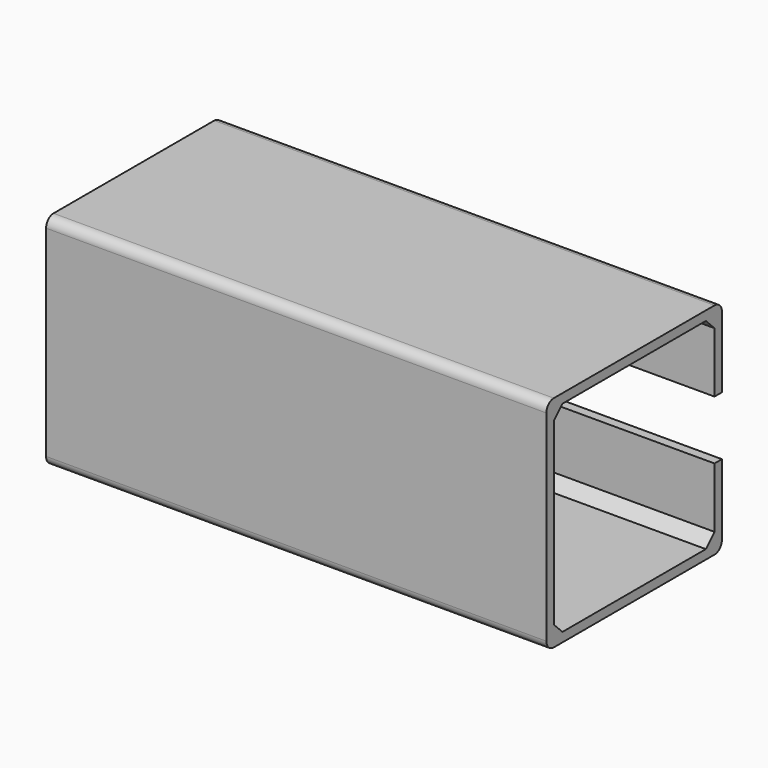
from build123d import *

# Parameters (mm, degrees)
F1_W      = 47.35
F1_H      = 47.35
F2_DEPTH  = 2
F3_DEPTH  = 107.95
F4_R      = 6.35
F7_DEPTH  = 107.951
F8_R      = 6.35
F9_DEPTH  = 25
F10_R     = 2
F11_W     = 2
F11_H     = 12.7
F12_DEPTH = 107.951
F13_DEPTH = 25


# Not quite as in the source:
# - a feature names something its author has since deleted; it is built from what else it names


with BuildPart() as f2:
    # F1 (on Right) → F2 (new body)
    with BuildSketch(Plane.YZ):
        Rectangle(F1_W, F1_H)
        Polygon((19.3428993274, 21.675), (21.675, 21.675), (21.675, 19.3428993274), (21.675, -19.3428993274), (21.675, -21.675), (19.3428993274, -21.675), (-19.3428993274, -21.675), (-21.675, -21.675), (-21.675, -19.3428993274), (-21.675, 19.3428993274), (-21.675, 21.675), (-19.3428993274, 21.675), align=None, mode=Mode.SUBTRACT)
        Polygon((21.675, 19.3428993274), (19.3428993274, 21.675), (-19.3428993274, 21.675), (-21.675, 19.3428993274), (-21.675, -19.3428993274), (-19.3428993274, -21.675), (19.3428993274, -21.675), (21.675, -19.3428993274), align=None)
        Polygon((-19.3428993274, -21.675), (-21.675, -19.3428993274), (-21.675, -21.675), align=None)
        Polygon((21.675, -21.675), (21.675, -19.3428993274), (19.3428993274, -21.675), align=None)
        Polygon((21.675, 19.3428993274), (21.675, 21.675), (19.3428993274, 21.675), align=None)
        Polygon((-21.675, 19.3428993274), (-19.3428993274, 21.675), (-21.675, 21.675), align=None)
    extrude(amount=F2_DEPTH)

    # F1 (on Right) → F3 (join)
    with BuildSketch(Plane.YZ):
        Rectangle(F1_W, F1_H)
        Polygon((19.3428993274, 21.675), (21.675, 21.675), (21.675, 19.3428993274), (21.675, -19.3428993274), (21.675, -21.675), (19.3428993274, -21.675), (-19.3428993274, -21.675), (-21.675, -21.675), (-21.675, -19.3428993274), (-21.675, 19.3428993274), (-21.675, 21.675), (-19.3428993274, 21.675), align=None, mode=Mode.SUBTRACT)
        Polygon((21.675, 19.3428993274), (21.675, 21.675), (19.3428993274, 21.675), align=None)
        Polygon((21.675, -21.675), (21.675, -19.3428993274), (19.3428993274, -21.675), align=None)
        Polygon((-19.3428993274, -21.675), (-21.675, -19.3428993274), (-21.675, -21.675), align=None)
        Polygon((-21.675, 19.3428993274), (-19.3428993274, 21.675), (-21.675, 21.675), align=None)
    extrude(amount=F3_DEPTH)

    # F4 (on face) → F7 (cut, through all)
    with BuildSketch(Plane.YZ):
        Circle(F4_R)
    extrude(amount=F7_DEPTH, mode=Mode.SUBTRACT)

    # F8 (on face) → F9 (cut)
    with BuildSketch(Plane(origin=(0, 23.675, 0), x_dir=(-1, 0, 0), z_dir=(0, 1, 0))):
        with Locations((-94.95, 0)):
            Circle(F8_R)
    extrude(amount=-F9_DEPTH, mode=Mode.SUBTRACT)

    # F10
    f10_edges = [f2.edges().sort_by_distance(p)[0] for p in [
        (53.975, -23.675, 23.675),
        (53.975, 23.675, 23.675),
        (53.975, 23.675, -23.675),
        (53.975, -23.675, -23.675),
    ]]
    fillet(f10_edges, radius=F10_R)

    # F11 (on face) → F12 (cut, through all)
    with BuildSketch(Plane.YZ.offset(107.95)):
        with Locations((22.675, 0)):
            Rectangle(F11_W, F11_H)
    extrude(amount=-F12_DEPTH, mode=Mode.SUBTRACT)

    # F1 (on Right) → F13 (cut)
    with BuildSketch(Plane.YZ):
        Polygon((21.675, 19.3428993274), (19.3428993274, 21.675), (-19.3428993274, 21.675), (-21.675, 19.3428993274), (-21.675, -19.3428993274), (-19.3428993274, -21.675), (19.3428993274, -21.675), (21.675, -19.3428993274), align=None)
    extrude(amount=F13_DEPTH, mode=Mode.SUBTRACT)


solid = f2.part
